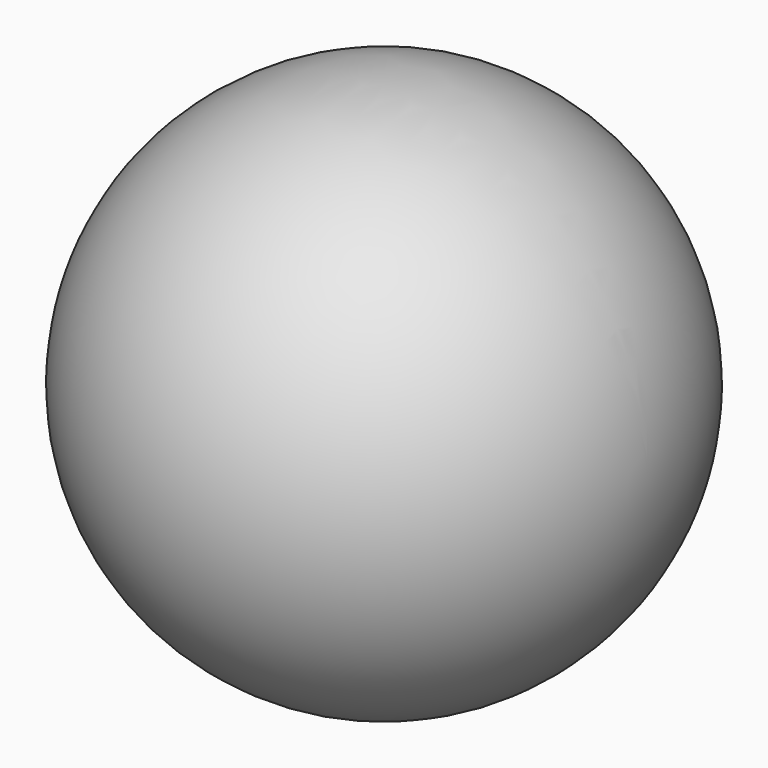
from build123d import *


with BuildPart() as f1:
    # F0 (on Front) → F1 (revolve)
    with BuildSketch(Plane.XZ):
        with BuildLine():
            Line((0, 0), (23.7865331613, 0))
            ThreePointArc((23.7865331613, 0), (0, 23.7865331613), (-23.7865331613, 0))
            Line((-23.7865331613, 0), (0, 0))
        make_face()
    revolve(axis=Axis((0, 0, 0), (1, 0, 0)))


solid = f1.part
